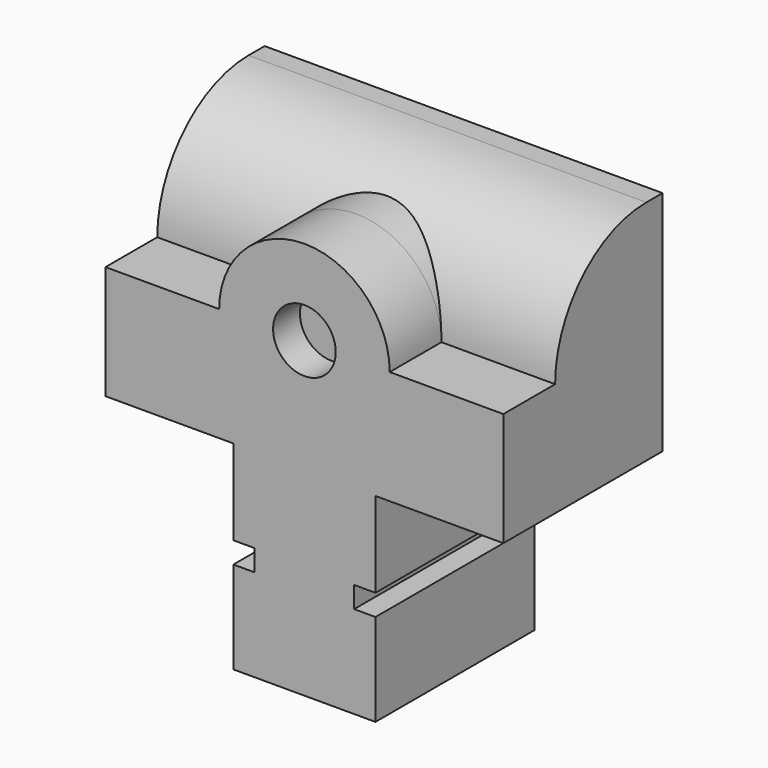
from build123d import *

# Parameters (mm, degrees)
F1_DEPTH    = 44.45
F2_W        = 30
F2_H        = 25.4
F3_DEPTH    = 88.9
F4_T4_DEPTH = 216.4
F4_S6_R     = 19.05
F4_T7_DEPTH = 111
F5_R        = 9.525
F6_DEPTH    = 12.7
F7_R        = 2
F8_DEPTH    = 5
F9_R        = 9.525
F10_DEPTH   = 24.5
F11_R       = 7
F12_DEPTH   = 7.5


# Not quite as in the source:
# - a fillet or chamfer that OpenCascade refuses, or shapes differently, is made with other operations: its cross-section is extruded or revolved along the edge and cut away or added


with BuildPart() as f1:
    # F0 (on Front) → F1 (new body)
    with BuildSketch(Plane.XZ):
        with BuildLine():
            Line((0, 0), (19.05, 0))
            ThreePointArc((19.05, 0), (0, 19.05), (-19.05, 0))
            Line((-19.05, 0), (0, 0))
        make_face()
        with BuildLine():
            Line((44.45, 0), (19.05, 0))
            ThreePointArc((19.05, 0), (0, -19.05), (-19.05, 0))
            Line((-19.05, 0), (-44.45, 0))
            Line((-44.45, 0), (-44.45, -25.4))
            Line((-44.45, -25.4), (-15.875, -25.4))
            Line((-15.875, -25.4), (-15.875, -44.45))
            Line((-15.875, -44.45), (-11.1125, -44.45))
            Line((-11.1125, -44.45), (-11.1125, -49.2125))
            Line((-11.1125, -49.2125), (-15.875, -49.2125))
            Line((-15.875, -49.2125), (-15.875, -69.85))
            Line((-15.875, -69.85), (15.875, -69.85))
            Line((15.875, -69.85), (15.875, -49.2125))
            Line((15.875, -49.2125), (11.1125, -49.2125))
            Line((11.1125, -49.2125), (11.1125, -44.45))
            Line((11.1125, -44.45), (15.875, -44.45))
            Line((15.875, -44.45), (15.875, -25.4))
            Line((15.875, -25.4), (44.45, -25.4))
            Line((44.45, -25.4), (44.45, 0))
        make_face()
        with BuildLine():
            ThreePointArc((-19.05, 0), (0, -19.05), (19.05, 0))
            Line((19.05, 0), (0, 0))
            Line((0, 0), (-19.05, 0))
        make_face()
    extrude(amount=F1_DEPTH)

    # F2 (on face) → F3 (join)
    with BuildSketch(Plane(origin=(-44.45, 0, 0), x_dir=(0, -1, 0), z_dir=(-1, 0, 0))):
        with Locations((15, 12.7)):
            Rectangle(F2_W, F2_H)
    extrude(amount=-F3_DEPTH)

    # F4: fillet of radius 25.5 on 1 edges, made by hand


with BuildPart() as f4_tool2:
    # F4_s3 → F4_t4 (new body)
    with BuildSketch(Plane.YZ.offset(-108.2)):
        with BuildLine():
            ThreePointArc((-30, -0.1), (-22.5312229203, 17.9312229203), (-4.5, 25.4))
            Line((-4.5, 25.4), (-30, 25.4))
            Line((-30, 25.4), (-30, -0.1))
        make_face()
    extrude(amount=F4_T4_DEPTH)

    split(bisect_by=Plane.XY, keep=Keep.TOP)

    # F4_s6 → F4_t7 (cut, symmetric)
    with BuildSketch(Plane.XZ.offset(17.2)):
        Circle(F4_S6_R)
    extrude(amount=F4_T7_DEPTH, both=True, mode=Mode.SUBTRACT)


with BuildPart() as f1_1:
    add(f1.part)

    # F4_t1: cut F4_tool2
    add(f4_tool2.part, mode=Mode.SUBTRACT)

    # F5 (on face) → F6 (cut)
    with BuildSketch(Plane.XZ.offset(44.45)):
        Circle(F5_R)
    extrude(amount=-F6_DEPTH, mode=Mode.SUBTRACT)

    # F7 (on face) → F8 (cut)
    with BuildSketch(Plane(origin=(0, 0, 0), x_dir=(-1, 0, 0), z_dir=(0, 1, 0))):
        with BuildLine():
            ThreePointArc((-27.45, 10.4), (-29.45, 12.4), (-31.45, 10.4))
            ThreePointArc((-31.45, 10.4), (-29.45, 8.4), (-27.45, 10.4))
        make_face()
        with Locations((29.45, 10.4)):
            Circle(F7_R)
    extrude(amount=-F8_DEPTH, mode=Mode.SUBTRACT)

    # F9 (on face) → F10 (join)
    with BuildSketch(Plane.XZ.offset(44.45)):
        Circle(F9_R)
    extrude(amount=-F10_DEPTH)

    # F11 (on face) → F12 (cut)
    with BuildSketch(Plane.XZ.offset(44.45)):
        Circle(F11_R)
    extrude(amount=-F12_DEPTH, mode=Mode.SUBTRACT)


solid = f1_1.part
